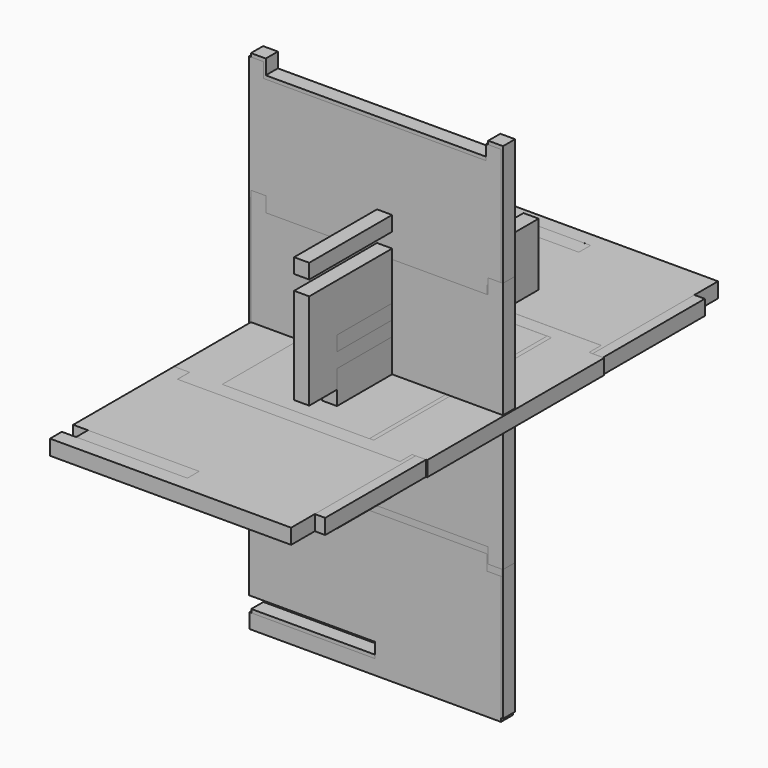
from build123d import *

# Parameters (mm, degrees)
F0_W      = 264.8
F0_H      = 17.7
F12_DEPTH = 18
F1_W      = 264.8
F1_H      = 17.7
F13_DEPTH = 18
F14_DEPTH = 18
F15_DEPTH = 18
F16_DEPTH = 18
F17_DEPTH = 18
F6_W      = 264
F6_H      = 17.7
F18_DEPTH = 18
F7_W      = 264
F7_H      = 17.7
F19_DEPTH = 18
F8_W      = 175
F8_H      = 264.4
F20_DEPTH = 18
F9_W      = 175
F9_H      = 264.4
F21_DEPTH = 18
F22_DEPTH = 18
F23_DEPTH = 18


# Not quite as in the source:
# - ends of sketch curves that miss each other by under 0.0002 mm in the source are joined


with BuildPart() as f12:
    # F0 (on Front) → F12 (new body)
    with BuildSketch(Plane.XZ):
        Polygon((-149.6062576771, -300), (150, -300), (150, 300), (132.4, 300), (132.4, 282.4), (-132.4, 282.4), (-132.4, 300), (-150, 300), (-149.7333943844, -264.8), (0, -264.8), (0, -282.4), (-149.6062576771, -282.4), align=None)
        Rectangle(F0_W, F0_H, mode=Mode.SUBTRACT)
    extrude(amount=F12_DEPTH)


with BuildPart() as f13:
    # F1 (on Front) → F13 (new body)
    with BuildSketch(Plane.XZ):
        Polygon((-152.021214366, -304.1411764706), (147.5850433111, -304.1411764706), (147.5850433111, 295.8588235294), (129.9850433111, 295.8588235294), (129.9850433111, 278.2588235294), (-134.8149566889, 278.2588235294), (-134.8149566889, 295.8588235294), (-152.4149566889, 295.8588235294), (-152.1483510733, -268.9411764706), (-2.4149566889, -268.9411764706), (-2.4149566889, -286.5411764706), (-152.021214366, -286.5411764706), align=None)
        with Locations((-2.4149566889, -4.1411764706)):
            Rectangle(F1_W, F1_H, mode=Mode.SUBTRACT)
    extrude(amount=F13_DEPTH)


with BuildPart() as f14:
    # F2 (on Top) → F14 (new body)
    with BuildSketch(Plane.XY):
        Polygon((132.385053514, -282.5411762625), (149.985053514, -282.5411762625), (149.985053514, 282.2588237375), (132.385053514, 282.2588237375), (132.385053514, 299.8588237375), (-132.414946486, 299.8588237375), (-132.414946486, 282.2588237375), (-150.014946486, 282.2588237375), (-150.014946486, 8.7088237375), (-132.414946486, 8.7088237375), (0, 8.7088237375), (0, -8.9911762625), (-132.414946486, -8.9911762625), (-150.014946486, -8.9911762625), (-150.014946486, -282.5411762625), (-132.414946486, -282.5411762625), (-132.414946486, -300.1411762625), (132.385053514, -300.1411762625), align=None)
    extrude(amount=F14_DEPTH)


with BuildPart() as f15:
    # F3 (on Top) → F15 (new body)
    with BuildSketch(Plane.XY):
        Polygon((-149.8627406966, 282.263140464), (-149.7336154024, 8.713140464), (0.1289514797, 8.713140464), (0, -8.986859536), (-149.7252564861, -8.9950985407), (-149.4773061974, -282.536859536), (0, -282.536859536), (0, -300.136859536), (-149.4773061974, -300.136859536), (-149.4773061974, -317.736859536), (137.6065164804, -317.736859536), (137.6065164804, 299.863140464), (137.6065164804, 317.463140464), (-149.8710485203, 317.463140464), (-149.8710485203, 299.863140464), (-0.0082744317, 299.863140464), (0, 282.3338809885), align=None)
    extrude(amount=F15_DEPTH)


with BuildPart() as f16:
    # F4 (on Top) → F16 (new body)
    with BuildSketch(Plane.XY):
        Polygon((-131.6689617634, -150.224139154), (133.1310382366, -150.224139154), (133.1310382366, -132.224139154), (151.1310382366, -132.224139154), (151.1310382366, 130.975860846), (133.1310382366, 130.975860846), (133.1310382366, 148.975860846), (-131.6689617634, 148.975860846), (-131.6689617634, 130.975860846), (-149.6689617634, 130.975860846), (-149.6689617634, 8.375860846), (0.3310382366, 8.375860846), (0.3310382366, -9.224139154), (-149.6689617634, -9.224139154), (-149.6689617634, -132.224139154), (-131.6689617634, -132.224139154), align=None)
    extrude(amount=F16_DEPTH)


with BuildPart() as f17:
    # F5 (on Top) → F17 (new body)
    with BuildSketch(Plane.XY):
        Polygon((-131.409532547, -150.428586483), (133.390467453, -150.428586483), (133.390467453, -132.428586483), (151.390467453, -132.428586483), (151.390467453, 130.771413517), (133.390467453, 130.771413517), (133.390467453, 148.771413517), (-131.409532547, 148.771413517), (-131.409532547, 130.771413517), (-149.409532547, 130.771413517), (-149.409532547, 8.171413517), (0.590467453, 8.171413517), (0.590467453, -9.428586483), (-149.409532547, -9.428586483), (-149.409532547, -132.428586483), (-131.409532547, -132.428586483), align=None)
    extrude(amount=F17_DEPTH)


with BuildPart() as f18:
    # F6 (on Front) → F18 (new body)
    with BuildSketch(Plane.XZ):
        Polygon((130.9714285714, -151.5714973211), (148.9714285714, -151.5714973211), (148.9714285714, 148.4285026789), (130.9714285714, 148.4285026789), (130.9714285714, 130.5785026789), (-133.0285714286, 130.5785026789), (-133.0285714286, 148.4285026789), (-151.0285714286, 148.4285026789), (-151.0285714286, -151.5714973211), (-133.0285714286, -151.5714973211), (-133.0285714286, -133.4214973211), (-1.0285714286, -133.4214973211), (130.9714285714, -133.4214973211), align=None)
        with Locations((-1.0285714286, -1.5714973211)):
            Rectangle(F6_W, F6_H, mode=Mode.SUBTRACT)
    extrude(amount=F18_DEPTH)


with BuildPart() as f19:
    # F7 (on Front) → F19 (new body)
    with BuildSketch(Plane.XZ):
        Polygon((132, -143.75), (150, -143.75), (150, 156.25), (132, 156.25), (132, 138.4), (-132, 138.4), (-132, 156.25), (-150, 156.25), (-150, -143.75), (-132, -143.75), (-132, -125.6), (0, -125.6), (132, -125.6), align=None)
        with Locations((0, 6.25)):
            Rectangle(F7_W, F7_H, mode=Mode.SUBTRACT)
    extrude(amount=F19_DEPTH)


with BuildPart() as f20:
    # F8 (on Top) → F20 (new body)
    with BuildSketch(Plane.XY):
        Rectangle(F8_W, F8_H)
    extrude(amount=F20_DEPTH)


with BuildPart() as f21:
    # F9 (on Top) → F21 (new body)
    with BuildSketch(Plane.XY):
        with Locations((-5.1, -0.2)):
            Rectangle(F9_W, F9_H)
    extrude(amount=F21_DEPTH)


with BuildPart() as f22:
    # F10 (on Right) → F22 (new body)
    with BuildSketch(Plane.YZ):
        Polygon((8.6638122797, 17.6), (-141.3361877203, 17.6), (-141.3361877203, 0), (158.6638122797, 0), (158.6638182402, 185), (-141.3361817598, 185), (-141.3361817598, 167.4), (8.6638182402, 167.4), (8.6638182402, 149.8), (-141.3361817598, 149.8), (-141.3361817598, 35.2739133894), (8.6638122797, 35.2), align=None)
    extrude(amount=F22_DEPTH)


with BuildPart() as f23:
    # F11 (on Right) → F23 (new body)
    with BuildSketch(Plane.YZ):
        Polygon((49.9999985099, -92.6978261158), (-100.0000014901, -92.6978261158), (-100.0000014901, -110.2978261158), (199.9999985099, -110.2978261158), (200.0000022352, 92.5021738842), (-99.9999977648, 92.5021738842), (-99.9999977648, 74.9021738842), (50.0000022352, 74.9021738842), (50.0000022352, 57.3021738842), (-99.9999977648, 57.3021738842), (-99.9999955297, -75.0239127263), (49.9999985099, -75.0978261158), align=None)
    extrude(amount=F23_DEPTH)


solid = Compound([f12.part, f13.part, f14.part, f15.part, f16.part, f17.part, f18.part, f19.part, f20.part, f21.part, f22.part, f23.part])
